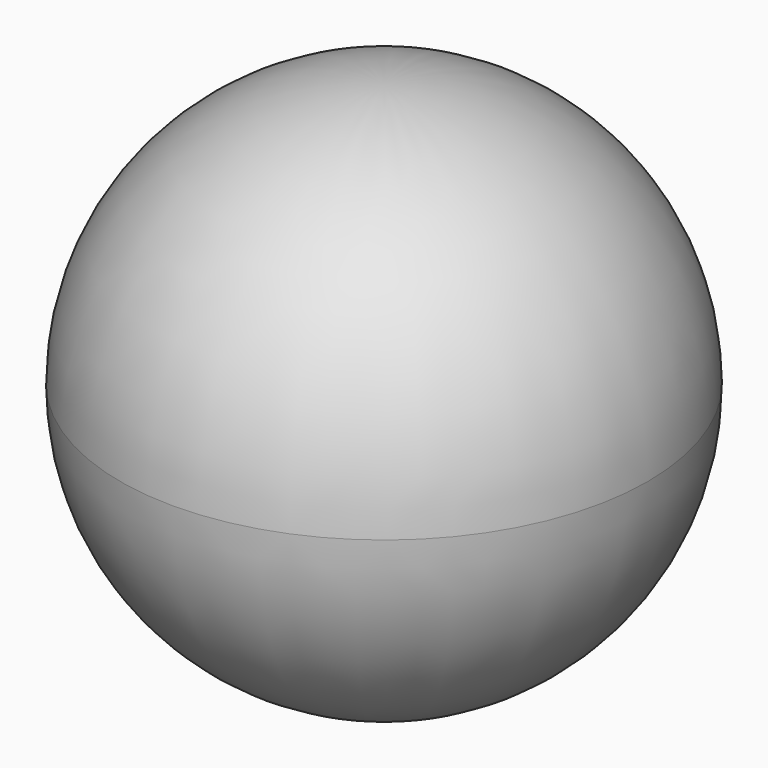
from build123d import *

# Parameters (mm, degrees)
F0_R          = 121.285
F1_DEPTH      = 121.285
F1_DEPTH_BACK = 121.285
F2_R          = 121.28499


# Not quite as in the source:
# - a fillet or chamfer is up to 0.001 mm smaller than in the source, because OpenCascade refuses the exact size


with BuildPart() as f1:
    # F0 (on Top) → F1 (new body, two sides)
    with BuildSketch(Plane.XY) as f1_sk:
        Circle(F0_R)
    extrude(amount=F1_DEPTH)
    extrude(f1_sk.sketch, amount=-F1_DEPTH_BACK)

    # F2 (radius 121.285 in the source; OpenCascade refuses exactly that, so slightly less here)
    f2_edges = [f1.edges().sort_by_distance(p)[0] for p in [
        (-121.285, 0, 121.285),
        (-121.285, 0, -121.285),
    ]]
    fillet(f2_edges, radius=F2_R)


solid = f1.part
